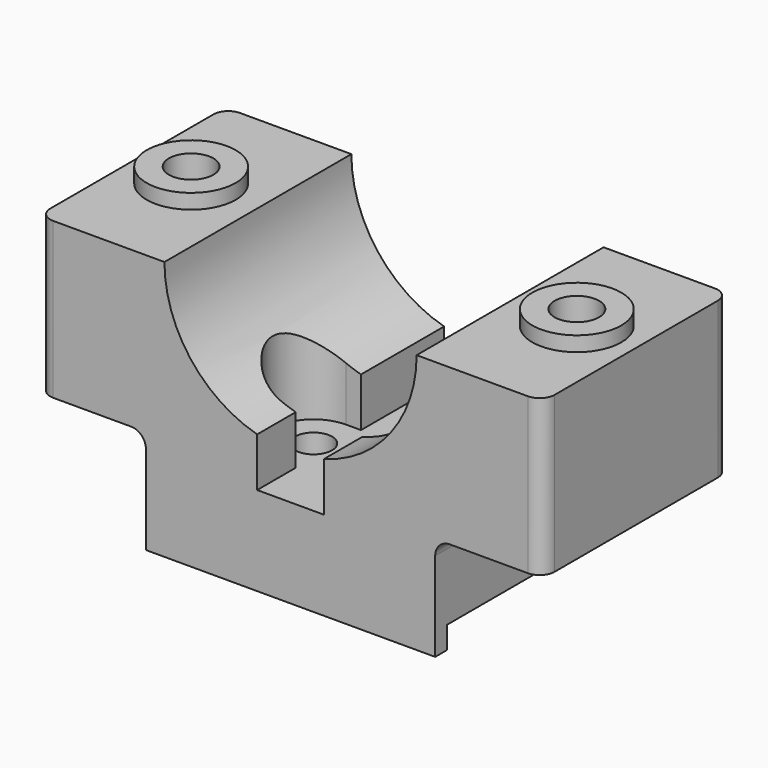
from build123d import *

# Parameters (mm, degrees)
F0_W      = 68
F0_H      = 31.5
F1_DEPTH  = 21
F2_W      = 39
F2_H      = 31.5
F3_DEPTH  = 11
F4_R      = 6
F5_DEPTH  = 2
F6_R      = 3
F7_DEPTH  = 34.001
F9_DEPTH  = 10
F11_DEPTH = 31.501
F12_W     = 39
F12_H     = 2
F13_DEPTH = 3
F14_R     = 2.5
F15_DEPTH = 34.001
F17_DEPTH = 25.001
F18_R     = 2
F19_R     = 1.99999


# Not quite as in the source:
# - a fillet or chamfer is up to 0.001 mm smaller than in the source, because OpenCascade refuses the exact size


with BuildPart() as f1:
    # F0 (on Top) → F1 (new body)
    with BuildSketch(Plane.XY):
        Rectangle(F0_W, F0_H)
    extrude(amount=-F1_DEPTH)

    # F2 (on face) → F3 (join)
    with BuildSketch(Plane(origin=(0, 0, -21), x_dir=(1, 0, 0), z_dir=(0, 0, -1))):
        Rectangle(F2_W, F2_H)
    extrude(amount=F3_DEPTH)

    # F4 (on face) → F5 (join)
    with BuildSketch(Plane.XY):
        with Locations((-26, 0)):
            Circle(F4_R)
        with Locations((26, 0)):
            Circle(F4_R)
    extrude(amount=F5_DEPTH)

    # F6 (on face) → F7 (cut, through all)
    with BuildSketch(Plane.XY.offset(2)):
        with Locations((-26, 0)):
            Circle(F6_R)
        with Locations((26, 0)):
            Circle(F6_R)
    extrude(amount=-F7_DEPTH, mode=Mode.SUBTRACT)

    # F8 (on face) → F9 (cut)
    with BuildSketch(Plane(origin=(0, 0, -21), x_dir=(1, 0, 0), z_dir=(0, 0, -1))):
        Polygon((-26, 5.1961524227), (-30.5, 2.5980762114), (-30.5, -2.5980762114), (-26, -5.1961524227), (-21.5, -2.5980762114), (-21.5, 2.5980762114), align=None)
        Polygon((26, -5.1961524227), (30.5, -2.5980762114), (30.5, 2.5980762114), (26, 5.1961524227), (21.5, 2.5980762114), (21.5, -2.5980762114), align=None)
    extrude(amount=-F9_DEPTH, mode=Mode.SUBTRACT)

    # F10 (on face) → F11 (cut, through all)
    with BuildSketch(Plane.XZ.offset(15.75)):
        with BuildLine():
            Line((4.5, -23), (4.5, -16.3935963108))
            ThreePointArc((4.5, -16.3935963108), (13.5185058346, -10.307764064), (17, 0))
            Line((17, 0), (-17, 0))
            ThreePointArc((-17, 0), (-13.5185058346, -10.307764064), (-4.5, -16.3935963108))
            Line((-4.5, -16.3935963108), (-4.5, -23))
            Line((-4.5, -23), (4.5, -23))
        make_face()
    extrude(amount=-F11_DEPTH, mode=Mode.SUBTRACT)

    # F12 (on face) → F13 (join)
    with BuildSketch(Plane(origin=(0, 0, -32), x_dir=(1, 0, 0), z_dir=(0, 0, -1))):
        with Locations((0, 14.75)):
            Rectangle(F12_W, F12_H)
    extrude(amount=F13_DEPTH)

    # F14 (on face) → F15 (cut, through all)
    with BuildSketch(Plane(origin=(0, 0, -32), x_dir=(1, 0, 0), z_dir=(0, 0, -1))):
        with Locations((-6.5, 3.7527767497)):
            Circle(F14_R)
        with Locations((6.5, 3.7527767497)):
            Circle(F14_R)
        with Locations((0, -7.5055534995)):
            Circle(F14_R)
    extrude(amount=-F15_DEPTH, mode=Mode.SUBTRACT)

    # F16 (on face) → F17 (cut, through all)
    with BuildSketch(Plane.XY.offset(-23)):
        with BuildLine():
            ThreePointArc((-6.5, 1.7472232503), (-12, -3.7527767497), (-6.5, -9.2527767497))
            Line((-6.5, -9.2527767497), (6.5, -9.2527767497))
            ThreePointArc((6.5, -9.2527767497), (12, -3.7527767497), (6.5, 1.7472232503))
            Line((6.5, 1.7472232503), (-6.5, 1.7472232503))
        make_face()
    extrude(amount=F17_DEPTH, mode=Mode.SUBTRACT)

    # F18
    f18_edges = [f1.edges().sort_by_distance(p)[0] for p in [
        (-34, -15.75, -10.5),
        (34, -15.75, -10.5),
        (34, 15.75, -10.5),
        (-34, 15.75, -10.5),
    ]]
    fillet(f18_edges, radius=F18_R)

    # F19 (radius 2 in the source; OpenCascade refuses exactly that, so slightly less here)
    f19_edges = [f1.edges().sort_by_distance(p)[0] for p in [
        (-19.5, 0, -21),
        (19.5, 0, -21),
    ]]
    fillet(f19_edges, radius=F19_R)


solid = f1.part
